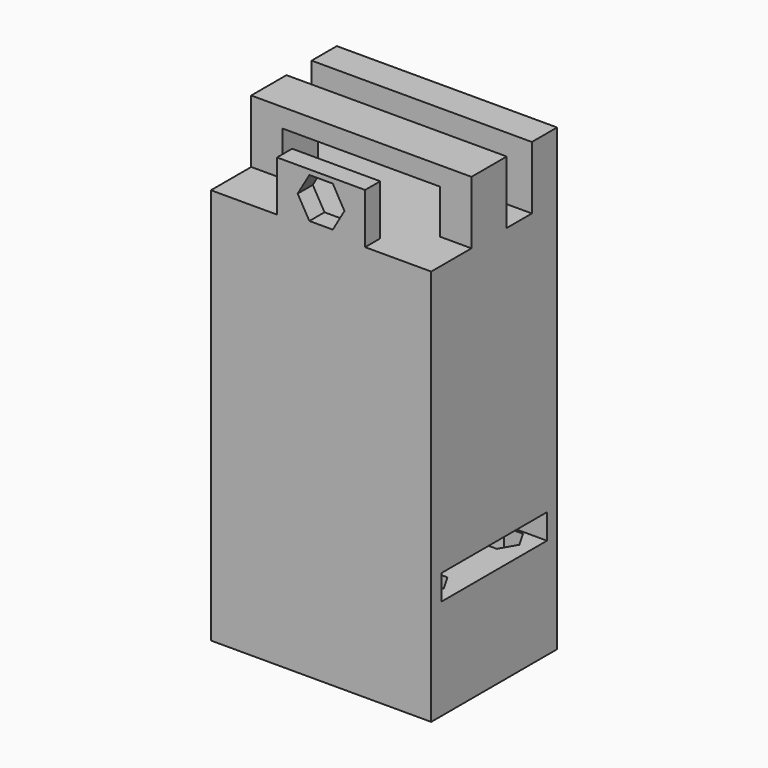
from build123d import *

# Parameters (mm, degrees)
F0_W      = 35
F0_H      = 25
F0_R      = 1.75
F1_DEPTH  = 40
F2_W      = 35
F2_H      = 25
F3_DEPTH  = 23
F4_W      = 35
F4_H      = 5
F5_DEPTH  = 10
F6_W      = 35
F6_H      = 7
F7_DEPTH  = 10
F8_W      = 25
F8_H      = 7
F9_DEPTH  = 7
F10_W     = 14
F10_H     = 3
F11_DEPTH = 8
F15_DEPTH = 8
F16_W     = 21
F16_H     = 4
F17_DEPTH = 9
F18_DEPTH = 3


# Not quite as in the source:
# - a pattern or mirror of a feature is missing from the dataset's text; its kind, count and spacing are read off the source's solid


with BuildPart() as f1:
    # F0 (on Top) → F1 (new body)
    with BuildSketch(Plane.XY):
        Rectangle(F0_W, F0_H)
        with Locations((-12.5, -7.5)):
            Circle(F0_R, mode=Mode.SUBTRACT)
        with Locations((12.5, -7.5)):
            Circle(F0_R, mode=Mode.SUBTRACT)
        with Locations((-12.5, 7.5)):
            Circle(F0_R, mode=Mode.SUBTRACT)
        with Locations((12.5, 7.5)):
            Circle(F0_R, mode=Mode.SUBTRACT)
    extrude(amount=F1_DEPTH)

    # F2 (on face) → F3 (join)
    with BuildSketch(Plane.XY.offset(40)):
        Rectangle(F2_W, F2_H)
    extrude(amount=F3_DEPTH)

    # F4 (on face) → F5 (join)
    with BuildSketch(Plane.XY.offset(63)):
        with Locations((0, 10)):
            Rectangle(F4_W, F4_H)
    extrude(amount=F5_DEPTH)

    # F6 (on face) → F7 (join)
    with BuildSketch(Plane.XY.offset(63)):
        with Locations((0, -1)):
            Rectangle(F6_W, F6_H)
    extrude(amount=F7_DEPTH)

    # F8 (on face) → F9 (cut)
    with BuildSketch(Plane.XZ.offset(4.5)):
        with Locations((0, 66.5)):
            Rectangle(F8_W, F8_H)
    extrude(amount=-F9_DEPTH, mode=Mode.SUBTRACT)

    # F10 (on face) → F11 (join)
    with BuildSketch(Plane.XY.offset(63)):
        with Locations((0, -11)):
            Rectangle(F10_W, F10_H)
    extrude(amount=F11_DEPTH)

    # F14 (on offset) → F15 (cut)
    with BuildSketch(Plane.XY.offset(20)):
        Polygon((14.0011106999, -10.1), (15.5022213998, -7.5), (14.0011106999, -4.9), (10.9988893001, -4.9), (9.4977786002, -7.5), (10.9988893001, -10.1), align=None)
        Polygon((10.9988893001, 10.1), (9.4977786002, 7.5), (10.9988893001, 4.9), (14.0011106999, 4.9), (15.5022213998, 7.5), (14.0011106999, 10.1), align=None)
        Polygon((-10.9988893001, 4.9), (-9.4977786002, 7.5), (-10.9988893001, 10.1), (-14.0011106999, 10.1), (-15.5022213998, 7.5), (-14.0011106999, 4.9), align=None)
        Polygon((-14.0011106999, -10.1), (-10.9988893001, -10.1), (-9.4977786002, -7.5), (-10.9988893001, -4.9), (-14.0011106999, -4.9), (-15.5022213998, -7.5), align=None)
    extrude(amount=-F15_DEPTH, mode=Mode.SUBTRACT)

    # F16 (on face) → F17 (cut)
    with BuildSketch(Plane.YZ.offset(17.5)):
        with Locations((0, 18)):
            Rectangle(F16_W, F16_H)
    f17 = extrude(amount=-F17_DEPTH, mode=Mode.SUBTRACT)

    # F17_copies: F17 across plane
    add(f17.mirror(Plane(origin=(0, 0, 0), x_dir=(0, 0, -1), z_dir=(-1, 0, 0))), mode=Mode.SUBTRACT)

    # F12 (on face) → F18 (cut)
    with BuildSketch(Plane.XZ.offset(12.5)):
        Polygon((3.7173565517, 67), (1.8586782759, 70.2193252087), (-1.8586782759, 70.2193252087), (-3.7173565517, 67), (-1.8586782759, 63.7806747913), (1.8586782759, 63.7806747913), align=None)
    extrude(amount=-F18_DEPTH, mode=Mode.SUBTRACT)


solid = f1.part
